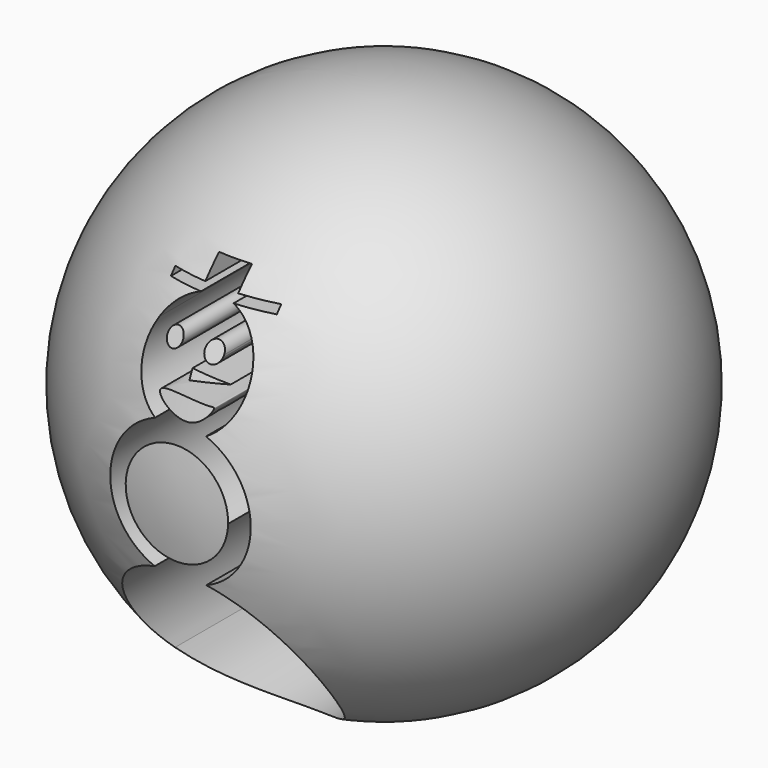
from build123d import *

# Parameters (mm, degrees)
F2_W     = 9.24971
F2_H     = 1.657442
F3_DEPTH = 63.5


with BuildPart() as f1:
    # F0 (on Front) → F1 (revolve)
    with BuildSketch(Plane.XZ):
        with BuildLine():
            Line((0, -64.731393), (0, 64.731393))
            ThreePointArc((0, 64.731393), (-64.731393, 0), (0, -64.731393))
        make_face()
    revolve(axis=Axis((0, 0, 0), (0, 0, -1)))

    # F2 (on Front) → F3 (cut, symmetric)
    with BuildSketch(Plane.XZ):
        with BuildLine():
            Line((3.984893, 39.496265), (-3.984893, 39.496265))
            ThreePointArc((-3.984893, 39.496265), (-8.409176, 36.994372), (-11.516483, 32.972135))
            Line((-11.516483, 32.972135), (-8.148138, 31.171527))
            ThreePointArc((-8.148138, 31.171527), (-6.104809, 33.214855), (-4.061481, 31.171527))
            Line((-4.061481, 31.171527), (1.47226, 31.171527))
            ThreePointArc((1.47226, 31.171527), (3.699886, 33.399153), (5.927512, 31.171527))
            ThreePointArc((5.927512, 31.171527), (5.909519, 30.888969), (5.855831, 30.610976))
            Line((5.855831, 30.610976), (11.050743, 33.831511))
            ThreePointArc((11.050743, 33.831511), (8.033676, 37.307336), (3.984893, 39.496265))
        make_face()
        Polygon((-3.984893, 41.153707), (-3.984893, 39.496265), (3.984893, 39.496265), (4.069874, 39.496265), (4.069874, 41.153707), (4.069874, 45.786072), (-3.984893, 45.786072), align=None)
        Polygon((-12.394612, 39.496265), (-3.984893, 39.496265), (-3.984893, 41.153707), (-12.468719, 41.153707), (-12.468719, 39.496265), align=None)
        with BuildLine():
            Line((-8.148138, 31.171527), (-11.516483, 32.972135))
            ThreePointArc((-11.516483, 32.972135), (-12.26033, 23.460623), (-6.238892, 16.060321))
            ThreePointArc((-6.238892, 16.060321), (0, 14.443199), (6.238892, 16.060321))
            ThreePointArc((6.238892, 16.060321), (12.397042, 23.929937), (11.050743, 33.831511))
            Line((11.050743, 33.831511), (5.855831, 30.610976))
            ThreePointArc((5.855831, 30.610976), (3.417328, 28.961894), (1.47226, 31.171527))
            Line((1.47226, 31.171527), (-4.061481, 31.171527))
            ThreePointArc((-4.061481, 31.171527), (-6.104809, 29.128198), (-8.148138, 31.171527))
        make_face()
        with BuildLine():
            add(Edge.make_bspline(
                [(-6.238892, 21.551825), (-5.563819, 22.905614), (5.429923, 21.342517), (7.641087, 22.156263), (2.781392, 14.618092), (-6.833287, 20.359827), (-6.238892, 21.551825)],
                knots=[0, 0, 0, 0, 0.340398, 0.453781, 0.700283, 1, 1, 1, 1], degree=3))
        make_face(mode=Mode.SUBTRACT)
        Polygon((9.064718, 26.54667), (0, 25.066717), (0, 27.286647), align=None, mode=Mode.SUBTRACT)
        with BuildLine():
            ThreePointArc((6.238892, 16.060321), (0, 14.443199), (-6.238892, 16.060321))
            ThreePointArc((-6.238892, 16.060321), (-17.22951, 0.040934), (-6.315133, -16.030496))
            ThreePointArc((-6.315133, -16.030496), (0, -17.229559), (6.315133, -16.030496))
            ThreePointArc((6.315133, -16.030496), (17.22951, 0.040934), (6.238892, 16.060321))
        make_face()
        with Locations((8.694729, 40.324986)):
            Rectangle(F2_W, F2_H)
        with BuildLine():
            ThreePointArc((6.315133, -16.030496), (0, -17.229559), (-6.315133, -16.030496))
            ThreePointArc((-6.315133, -16.030496), (-20.756269, -28.647961), (-20.380454, -47.821004))
            ThreePointArc((-20.380454, -47.821004), (0, -60.528382), (20.380454, -47.821004))
            ThreePointArc((20.380454, -47.821004), (20.756269, -28.647961), (6.315133, -16.030496))
        make_face()
    extrude(amount=F3_DEPTH, both=True, mode=Mode.SUBTRACT)


solid = f1.part
